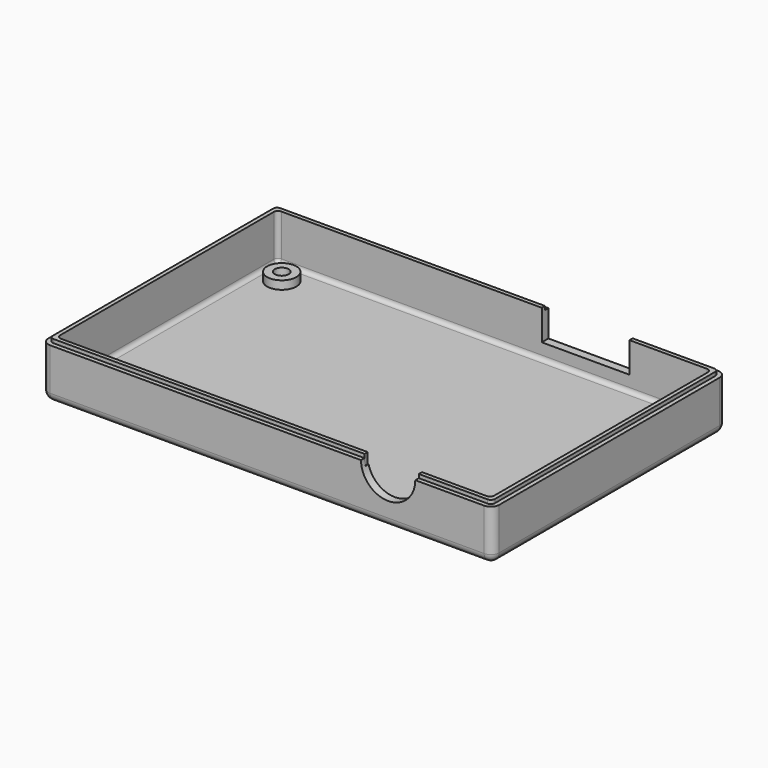
from build123d import *

# Parameters (mm, degrees)
F0_W           = 104
F0_H           = 66
F0_R           = 3
F1_DEPTH       = 2
F2_DEPTH       = 10.99
F3_DEPTH       = 10.1
F4_R           = 3.5
F5_DEPTH       = 2
F7_D           = 3.302
F7_CSINK_D     = 6.477
F7_CSINK_ANGLE = 82
F8_W           = 21
F8_H           = 6.4
F9_DEPTH       = 2.5
F10_W          = 13
F10_H          = 0.95
F11_DEPTH      = 2.5
F13_DEPTH      = 2.5
F14_R          = 2
F15_R          = 1
F16_W          = 21
F16_H          = 0.89
F17_DEPTH      = 2.5


# Not quite as in the source:
# - a feature names something its author has since deleted; it is built from what else it names


with BuildPart() as f1:
    # F0 (on Top) → F1 (new body)
    with BuildSketch(Plane.XY):
        with BuildLine():
            Line((61.6408709802, 21.8759292028), (-42.3591290198, 21.8759292028))
            ThreePointArc((-42.3591290198, 21.8759292028), (-43.7733425821, 21.2901427652), (-44.3591290198, 19.8759292028))
            Line((-44.3591290198, 19.8759292028), (-44.3591290198, -46.1240707972))
            ThreePointArc((-44.3591290198, -46.1240707972), (-43.7733425821, -47.5382843595), (-42.3591290198, -48.1240707972))
            Line((-42.3591290198, -48.1240707972), (61.6408709802, -48.1240707972))
            ThreePointArc((61.6408709802, -48.1240707972), (63.0550845426, -47.5382843595), (63.6408709802, -46.1240707972))
            Line((63.6408709802, -46.1240707972), (63.6408709802, 19.8759292028))
            ThreePointArc((63.6408709802, 19.8759292028), (63.0550845426, 21.2901427652), (61.6408709802, 21.8759292028))
        make_face()
        with BuildLine():
            ThreePointArc((-43.3091290198, 19.8759292028), (-43.0308804619, 20.547680645), (-42.3591290198, 20.8259292028))
            Line((-42.3591290198, 20.8259292028), (61.6408709802, 20.8259292028))
            ThreePointArc((61.6408709802, 20.8259292028), (62.3126224224, 20.547680645), (62.5908709802, 19.8759292028))
            Line((62.5908709802, 19.8759292028), (62.5908709802, -46.1240707972))
            ThreePointArc((62.5908709802, -46.1240707972), (62.3126224224, -46.7958222393), (61.6408709802, -47.0740707972))
            Line((61.6408709802, -47.0740707972), (-42.3591290198, -47.0740707972))
            ThreePointArc((-42.3591290198, -47.0740707972), (-43.0308804619, -46.7958222393), (-43.3091290198, -46.1240707972))
            Line((-43.3091290198, -46.1240707972), (-43.3091290198, 19.8759292028))
        make_face(mode=Mode.SUBTRACT)
        with BuildLine():
            Line((61.6408709802, 20.8259292028), (-42.3591290198, 20.8259292028))
            ThreePointArc((-42.3591290198, 20.8259292028), (-43.0308804619, 20.547680645), (-43.3091290198, 19.8759292028))
            Line((-43.3091290198, 19.8759292028), (-43.3091290198, -46.1240707972))
            ThreePointArc((-43.3091290198, -46.1240707972), (-43.0308804619, -46.7958222393), (-42.3591290198, -47.0740707972))
            Line((-42.3591290198, -47.0740707972), (61.6408709802, -47.0740707972))
            ThreePointArc((61.6408709802, -47.0740707972), (62.3126224224, -46.7958222393), (62.5908709802, -46.1240707972))
            Line((62.5908709802, -46.1240707972), (62.5908709802, 19.8759292028))
            ThreePointArc((62.5908709802, 19.8759292028), (62.3126224224, 20.547680645), (61.6408709802, 20.8259292028))
        make_face()
        with Locations((9.6408709802, -13.1240707972)):
            Rectangle(F0_W, F0_H, mode=Mode.SUBTRACT)
        with Locations((9.6408709802, -13.1240707972)):
            Rectangle(F0_W, F0_H)
        with Locations((-36.8591290198, -40.6240707972)):
            Circle(F0_R, mode=Mode.SUBTRACT)
        with Locations((57.1408709802, -40.6240707972)):
            Circle(F0_R, mode=Mode.SUBTRACT)
        with Locations((-36.8591290198, 14.3759292028)):
            Circle(F0_R, mode=Mode.SUBTRACT)
        with Locations((57.1408709802, 14.3759292028)):
            Circle(F0_R, mode=Mode.SUBTRACT)
        with Locations((-36.8591290198, -40.6240707972)):
            Circle(F0_R)
        with Locations((57.1408709802, -40.6240707972)):
            Circle(F0_R)
        with Locations((-36.8591290198, 14.3759292028)):
            Circle(F0_R)
        with Locations((57.1408709802, 14.3759292028)):
            Circle(F0_R)
    extrude(amount=-F1_DEPTH)

    # F0 (on Top) → F2 (join)
    with BuildSketch(Plane.XY):
        with BuildLine():
            Line((61.6408709802, 20.8259292028), (-42.3591290198, 20.8259292028))
            ThreePointArc((-42.3591290198, 20.8259292028), (-43.0308804619, 20.547680645), (-43.3091290198, 19.8759292028))
            Line((-43.3091290198, 19.8759292028), (-43.3091290198, -46.1240707972))
            ThreePointArc((-43.3091290198, -46.1240707972), (-43.0308804619, -46.7958222393), (-42.3591290198, -47.0740707972))
            Line((-42.3591290198, -47.0740707972), (61.6408709802, -47.0740707972))
            ThreePointArc((61.6408709802, -47.0740707972), (62.3126224224, -46.7958222393), (62.5908709802, -46.1240707972))
            Line((62.5908709802, -46.1240707972), (62.5908709802, 19.8759292028))
            ThreePointArc((62.5908709802, 19.8759292028), (62.3126224224, 20.547680645), (61.6408709802, 20.8259292028))
        make_face()
        with Locations((9.6408709802, -13.1240707972)):
            Rectangle(F0_W, F0_H, mode=Mode.SUBTRACT)
    extrude(amount=F2_DEPTH)

    # F0 (on Top) → F3 (join)
    with BuildSketch(Plane.XY):
        with BuildLine():
            Line((61.6408709802, 21.8759292028), (-42.3591290198, 21.8759292028))
            ThreePointArc((-42.3591290198, 21.8759292028), (-43.7733425821, 21.2901427652), (-44.3591290198, 19.8759292028))
            Line((-44.3591290198, 19.8759292028), (-44.3591290198, -46.1240707972))
            ThreePointArc((-44.3591290198, -46.1240707972), (-43.7733425821, -47.5382843595), (-42.3591290198, -48.1240707972))
            Line((-42.3591290198, -48.1240707972), (61.6408709802, -48.1240707972))
            ThreePointArc((61.6408709802, -48.1240707972), (63.0550845426, -47.5382843595), (63.6408709802, -46.1240707972))
            Line((63.6408709802, -46.1240707972), (63.6408709802, 19.8759292028))
            ThreePointArc((63.6408709802, 19.8759292028), (63.0550845426, 21.2901427652), (61.6408709802, 21.8759292028))
        make_face()
        with BuildLine():
            ThreePointArc((-43.3091290198, 19.8759292028), (-43.0308804619, 20.547680645), (-42.3591290198, 20.8259292028))
            Line((-42.3591290198, 20.8259292028), (61.6408709802, 20.8259292028))
            ThreePointArc((61.6408709802, 20.8259292028), (62.3126224224, 20.547680645), (62.5908709802, 19.8759292028))
            Line((62.5908709802, 19.8759292028), (62.5908709802, -46.1240707972))
            ThreePointArc((62.5908709802, -46.1240707972), (62.3126224224, -46.7958222393), (61.6408709802, -47.0740707972))
            Line((61.6408709802, -47.0740707972), (-42.3591290198, -47.0740707972))
            ThreePointArc((-42.3591290198, -47.0740707972), (-43.0308804619, -46.7958222393), (-43.3091290198, -46.1240707972))
            Line((-43.3091290198, -46.1240707972), (-43.3091290198, 19.8759292028))
        make_face(mode=Mode.SUBTRACT)
    extrude(amount=F3_DEPTH)

    # F4 (on face) → F5 (join)
    with BuildSketch(Plane.XY):
        with Locations((-36.8591290198, 14.3759292028)):
            Circle(F4_R)
        with Locations((56.1408709802, 14.3759292028)):
            Circle(F4_R)
        with Locations((56.1408709802, -40.6240707972)):
            Circle(F4_R)
        with Locations((-36.8591290198, -40.6240707972)):
            Circle(F4_R)
    extrude(amount=F5_DEPTH)

    # F7 (through all)
    with Locations(Plane(origin=(0, 0, -2), x_dir=(1, 0, 0), z_dir=(0, 0, -1))):
        with Locations((-36.8591290198, 40.6240707972), (56.1408709802, 40.6240707972), (56.1408709802, -14.3759292028), (-36.8591290198, -14.3759292028)):
            CounterSinkHole(F7_D / 2, F7_CSINK_D / 2, counter_sink_angle=F7_CSINK_ANGLE)

    # F8 (on face) → F9 (cut)
    with BuildSketch(Plane(origin=(0, 21.8759292028, 0), x_dir=(-1, 0, 0), z_dir=(0, 1, 0))):
        with Locations((-31.5408709802, 6.9)):
            Rectangle(F8_W, F8_H)
    extrude(amount=-F9_DEPTH, mode=Mode.SUBTRACT)

    # F10 (on face) → F11 (cut)
    with BuildSketch(Plane.XY.offset(10.99)):
        with Locations((38.6408709802, -46.5990707972)):
            Rectangle(F10_W, F10_H)
    extrude(amount=-F11_DEPTH, mode=Mode.SUBTRACT)

    # F12 (on face) → F13 (cut)
    with BuildSketch(Plane.XZ.offset(48.1240707972)):
        with BuildLine():
            ThreePointArc((32.1408709802, 10.1), (38.6408709802, 3.6), (45.1408709802, 10.1))
            Line((45.1408709802, 10.1), (32.1408709802, 10.1))
        make_face()
    extrude(amount=-F13_DEPTH, mode=Mode.SUBTRACT)

    # F14
    f14_edges = [f1.edges().sort_by_distance(p)[0] for p in [
        (63.640871, -13.124071, -2),
        (9.640871, 21.875929, -2),
        (-44.359129, -13.124071, -2),
        (9.640871, -48.124071, -2),
        (63.055085, 21.290143, -2),
        (-43.773343, 21.290143, -2),
        (63.055085, -47.538284, -2),
        (-43.773343, -47.538284, -2),
    ]]
    fillet(f14_edges, radius=F14_R)

    # F15
    f15_edges = [f1.edges().sort_by_distance(p)[0] for p in [
        (9.640871, 19.875929, 0),
        (-42.359129, 19.875929, 5.495),
        (-42.359129, -13.124071, 0),
        (9.640871, -46.124071, 0),
        (-42.359129, -46.124071, 5.495),
        (61.640871, 19.875929, 5.495),
        (61.640871, -13.124071, 0),
        (61.640871, -46.124071, 5.495),
    ]]
    fillet(f15_edges, radius=F15_R)

    # F16 (on face) → F17 (cut)
    with BuildSketch(Plane(origin=(0, 20.8259292028, 0), x_dir=(-1, 0, 0), z_dir=(0, 1, 0))):
        with Locations((-31.5408709802, 10.545)):
            Rectangle(F16_W, F16_H)
    extrude(amount=-F17_DEPTH, mode=Mode.SUBTRACT)


solid = f1.part
